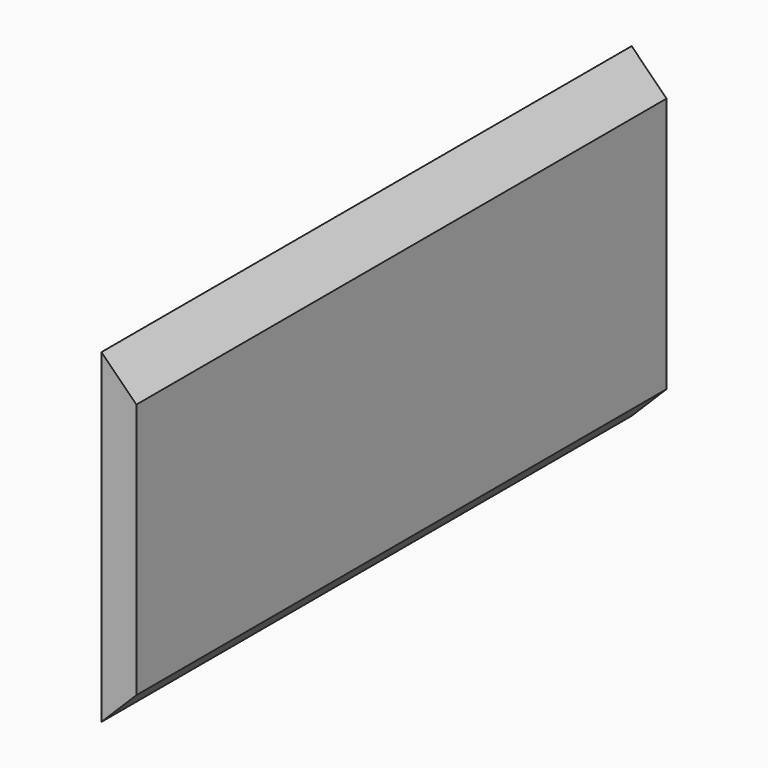
from build123d import *

# Parameters (mm, degrees)
F0_W     = 361.95
F0_H     = 177.8
F1_DEPTH = 19.05
F2_SIZE  = 19.04999


# Not quite as in the source:
# - a fillet or chamfer is up to 0.001 mm smaller than in the source, because OpenCascade refuses the exact size


with BuildPart() as f1:
    # F0 (on Right) → F1 (new body)
    with BuildSketch(Plane.YZ):
        Rectangle(F0_W, F0_H)
    extrude(amount=F1_DEPTH)

    # F2 (size 19.05 in the source; OpenCascade refuses exactly that, so slightly less here)
    f2_edges = [f1.edges().sort_by_distance(p)[0] for p in [
        (19.05, 0, 88.9),
        (19.05, 0, -88.9),
    ]]
    chamfer(f2_edges, length=F2_SIZE)


solid = f1.part
